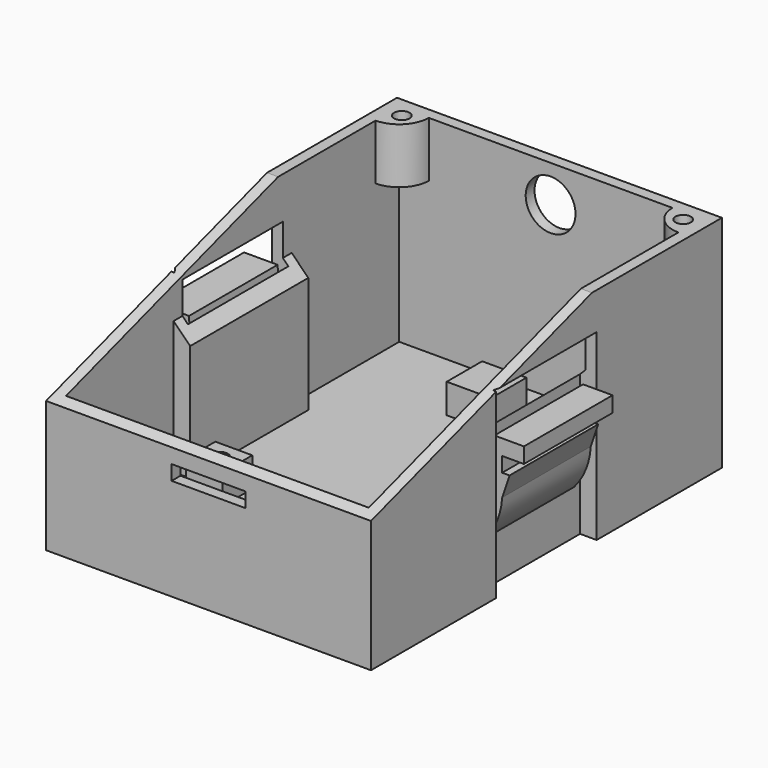
from build123d import *

# Parameters (mm, degrees)
F0_W      = 4
F0_H      = 17
F1_DEPTH  = 1.8
F3_DEPTH  = 22
F4_W      = 44
F4_H      = 59.4
F5_DEPTH  = 6
F6_W      = 2.25
F6_H      = 20
F7_DEPTH  = 10
F9_DEPTH  = 20
F11_DEPTH = 17
F13_DEPTH = 20
F15_DEPTH = 17
F17_DEPTH = 45
F18_R     = 3.375
F19_DEPTH = 3
F20_R     = 1.05
F21_DEPTH = 7.5
F22_W     = 10
F22_H     = 2
F23_DEPTH = 2.5
F25_START = 1
F24_W     = 2.95
F24_H     = 2.1
F25_DEPTH = 15
F26_W     = 5
F26_H     = 5
F26_R     = 1.2
F26_W_2   = 6
F26_H_2   = 6
F27_DEPTH = 4


# Not quite as in the source:
# - a feature names something its author has since deleted; it is built from what else it names


with BuildPart() as f1:
    # F0 (on Top) → F1 (new body)
    with BuildSketch(Plane.XY):
        Polygon((-12.630645159, 54.2783500865), (-56.630645159, 54.2783500865), (-56.630645159, 33.0783500865), (-54.380645159, 33.0783500865), (-54.380645159, 16.0783500865), (-56.630645159, 16.0783500865), (-56.630645159, -5.1216499135), (-12.630645159, -5.1216499135), (-12.630645159, 16.0783500865), (-14.880645159, 16.0783500865), (-14.880645159, 33.0783500865), (-12.630645159, 33.0783500865), align=None)
        with Locations((-18.730645159, 4.8783500865)):
            Rectangle(F0_W, F0_H, mode=Mode.SUBTRACT)
    extrude(amount=F1_DEPTH)

    # F2 (on face) → F3 (join)
    with BuildSketch(Plane.XY.offset(1.8)):
        Polygon((-12.630645159, 33.0783500865), (-12.630645159, 54.2783500865), (-56.630645159, 54.2783500865), (-56.630645159, 33.0783500865), (-54.380645159, 33.0783500865), (-54.380645159, 16.0783500865), (-56.630645159, 16.0783500865), (-56.630645159, -5.1216499135), (-12.630645159, -5.1216499135), (-12.630645159, 16.0783500865), (-14.880645159, 16.0783500865), (-14.880645159, 33.0783500865), align=None)
        Polygon((-55.130645159, 34.5783500865), (-55.130645159, 52.7783500865), (-14.130645159, 52.7783500865), (-14.130645159, 34.5783500865), (-16.380645159, 34.5783500865), (-16.380645159, 14.5783500865), (-14.130645159, 14.5783500865), (-14.130645159, -3.6216499135), (-16.730645159, -3.6216499135), (-20.730645159, -3.6216499135), (-55.130645159, -3.6216499135), (-55.130645159, 14.5783500865), (-52.880645159, 14.5783500865), (-52.880645159, 34.5783500865), align=None, mode=Mode.SUBTRACT)
    extrude(amount=F3_DEPTH)

    # F4 (on face) → F5 (join)
    with BuildSketch(Plane.XY.offset(23.8)):
        with Locations((-34.630645159, 24.5783500865)):
            Rectangle(F4_W, F4_H)
        Polygon((-55.130645159, 34.5783500865), (-55.130645159, 52.7783500865), (-14.130645159, 52.7783500865), (-14.130645159, 34.5783500865), (-16.380645159, 34.5783500865), (-16.380645159, 14.5783500865), (-14.130645159, 14.5783500865), (-14.130645159, -3.6216499135), (-55.130645159, -3.6216499135), (-55.130645159, 14.5783500865), (-52.880645159, 14.5783500865), (-52.880645159, 34.5783500865), align=None, mode=Mode.SUBTRACT)
    extrude(amount=F5_DEPTH)

    # F6 (on face) → F7 (cut)
    with BuildSketch(Plane.XY.offset(29.8)):
        with Locations((-54.005645159, 24.5783500865)):
            Rectangle(F6_W, F6_H)
        with Locations((-15.255645159, 24.5783500865)):
            Rectangle(F6_W, F6_H)
    extrude(amount=-F7_DEPTH, mode=Mode.SUBTRACT)

    # F8 (on face) → F9 (cut)
    with BuildSketch(Plane.XZ.offset(-14.5783500865)):
        Polygon((-52.880645159, 19.8), (-55.130645159, 19.8), (-52.880645159, 17.55), align=None)
    extrude(amount=-F9_DEPTH, mode=Mode.SUBTRACT)

    # F10 (on face) → F11 (cut)
    with BuildSketch(Plane.XZ.offset(-33.0783500865)):
        Polygon((-56.630645159, 24.8), (-56.630645159, 23.8), (-55.880645159, 23.8), (-54.380645159, 23.8), align=None)
    extrude(amount=F11_DEPTH, mode=Mode.SUBTRACT)

    # F12 (on face) → F13 (cut)
    with BuildSketch(Plane(origin=(0, 34.5783500865, 0), x_dir=(-1, 0, 0), z_dir=(0, 1, 0))):
        Polygon((16.380645159, 17.55), (16.380645159, 19.8), (14.130645159, 19.8), align=None)
    extrude(amount=-F13_DEPTH, mode=Mode.SUBTRACT)

    # F14 (on face) → F15 (cut)
    with BuildSketch(Plane(origin=(0, 16.0783500865, 0), x_dir=(-1, 0, 0), z_dir=(0, 1, 0))):
        Polygon((12.630645159, 24.8), (12.630645159, 23.8), (14.880645159, 23.8), align=None)
    extrude(amount=F15_DEPTH, mode=Mode.SUBTRACT)

    # F16 (on face) → F17 (cut)
    with BuildSketch(Plane.YZ.offset(-12.630645159)):
        Polygon((32.2783500865, 29.8), (-5.1216499135, 29.8), (-5.1216499135, 17.8), align=None)
    extrude(amount=-F17_DEPTH, mode=Mode.SUBTRACT)

    # F18 (on face) → F19 (cut)
    with BuildSketch(Plane(origin=(0, 54.2783500865, 0), x_dir=(-1, 0, 0), z_dir=(0, 1, 0))):
        with Locations((34.630645159, 24.8)):
            Circle(F18_R)
    extrude(amount=-F19_DEPTH, mode=Mode.SUBTRACT)

    # F20 (on face) → F21 (join)
    with BuildSketch(Plane.XY.offset(29.8)):
        with BuildLine():
            Line((-55.130645159, 52.7783500865), (-55.130645159, 48.7783500865))
            ThreePointArc((-55.130645159, 48.7783500865), (-52.3091414621, 49.9568463896), (-51.130645159, 52.7783500865))
            Line((-51.130645159, 52.7783500865), (-55.130645159, 52.7783500865))
        make_face()
        with Locations((-53.6807930499, 51.4078039413)):
            Circle(F20_R, mode=Mode.SUBTRACT)
        with BuildLine():
            Line((-14.130645159, 52.7783500865), (-18.130645159, 52.7783500865))
            ThreePointArc((-18.130645159, 52.7783500865), (-16.952148856, 49.9568463896), (-14.130645159, 48.7783500865))
            Line((-14.130645159, 48.7783500865), (-14.130645159, 52.7783500865))
        make_face()
        with Locations((-15.5804972681, 51.4078039413)):
            Circle(F20_R, mode=Mode.SUBTRACT)
    extrude(amount=-F21_DEPTH)

    # F22 (on face) → F23 (cut)
    with BuildSketch(Plane.XZ.offset(5.1216499135)):
        with Locations((-34.630645159, 14.8)):
            Rectangle(F22_W, F22_H)
    extrude(amount=-F23_DEPTH, mode=Mode.SUBTRACT)

    # F24 (on face) → F25 (join)
    with BuildSketch(Plane.XZ.offset(-33.0783500865).offset(F25_START)):
        with Locations((-11.155645159, 17.575)):
            Rectangle(F24_W, F24_H)
        with BuildLine():
            Line((-14.880645159, 9.525), (-14.880645159, 6))
            ThreePointArc((-14.880645159, 6), (-13.2978940887, 8.5959050075), (-12.630645159, 11.5621488653))
            Line((-12.630645159, 11.5621488653), (-12.630645159, 14.525))
            Line((-12.630645159, 14.525), (-12.630645159, 16.525))
            Line((-12.630645159, 16.525), (-12.630645159, 18.625))
            Line((-12.630645159, 18.625), (-13.680645159, 18.625))
            Line((-13.680645159, 18.625), (-14.880645159, 9.525))
        make_face()
        Polygon((-12.630645159, 14.525), (-12.630645159, 11.5621488653), (-11.630645159, 14.525), align=None)
        with BuildLine():
            Line((-57.630645159, 14.525), (-56.630645159, 11.5621488653))
            ThreePointArc((-56.630645159, 11.5621488653), (-55.9633962294, 8.5959050075), (-54.380645159, 6))
            Line((-54.380645159, 6), (-54.380645159, 8.2336284751))
            Line((-54.380645159, 8.2336284751), (-55.0399858184, 19.425))
            Line((-55.0399858184, 19.425), (-59.580645159, 19.425))
            Line((-59.580645159, 19.425), (-59.580645159, 17.325))
            Line((-59.580645159, 17.325), (-57.0257989239, 16.632160343))
            Line((-57.0257989239, 16.632160343), (-56.630645159, 15.525))
            Line((-56.630645159, 15.525), (-56.630645159, 14.525))
            Line((-56.630645159, 14.525), (-57.630645159, 14.525))
        make_face()
    extrude(amount=F25_DEPTH)

    # F26 (on face) → F27 (join)
    with BuildSketch(Plane.XY.offset(1.8)):
        with Locations((-48.730645159, 14.2783500865)):
            Rectangle(F26_W, F26_H)
        with Locations((-48.730645159, 14.2783500865)):
            Circle(F26_R, mode=Mode.SUBTRACT)
        with Locations((-26.330645159, 0.0783500865)):
            Rectangle(F26_W, F26_H)
        with Locations((-26.330645159, 0.0783500865)):
            Circle(F26_R, mode=Mode.SUBTRACT)
        with Locations((-17.130645159, 45.7783500865)):
            Rectangle(F26_W_2, F26_H_2)
        with Locations((-17.130645159, 45.7783500865)):
            Circle(F26_R, mode=Mode.SUBTRACT)
        with Locations((-37.6969575882, 45.7783500865)):
            Rectangle(F26_W_2, F26_H_2)
    extrude(amount=F27_DEPTH)


solid = f1.part
